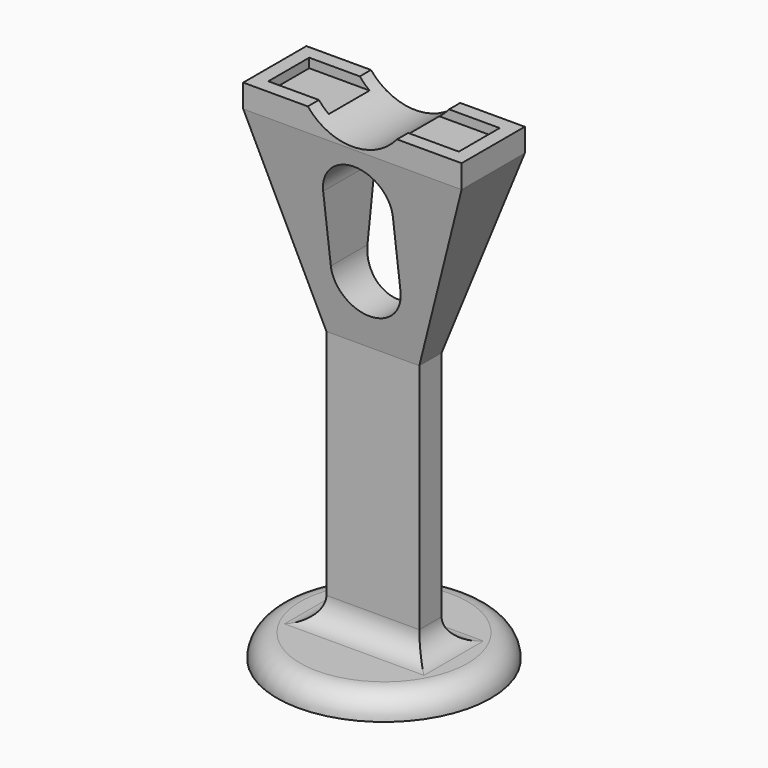
from build123d import *

# Parameters (mm, degrees)
F1_W       = 41
F1_H       = 11
F2_DEPTH   = 3
F1_W_2     = 47
F1_H_2     = 17
F3_DEPTH   = 5
F5_DEPTH   = 17.001
F6_R       = 23
F7_DEPTH   = 5
F8_W       = 20
F8_H       = 6
F9_DEPTH   = 55
F9_FACE_W  = 20
F9_FACE_H  = 6
F3_FACE1_W = 47
F3_FACE1_H = 17
F12_DEPTH  = 25
F13_R      = 4.99999


# Not quite as in the source:
# - a fillet or chamfer is up to 0.001 mm smaller than in the source, because OpenCascade refuses the exact size


with BuildPart() as f2:
    # F1 (on offset) → F2 (new body)
    with BuildSketch(Plane.XY.offset(100)):
        Rectangle(F1_W, F1_H)
    extrude(amount=F2_DEPTH)

    # F1 (on offset) → F3 (join)
    with BuildSketch(Plane.XY.offset(100)):
        Rectangle(F1_W_2, F1_H_2)
        Rectangle(F1_W, F1_H, mode=Mode.SUBTRACT)
    extrude(amount=F3_DEPTH)

    # F4 (on face) → F5 (cut, through all)
    with BuildSketch(Plane.XZ.offset(8.5)):
        with BuildLine():
            Line((9.6046863561, 105), (-9.6046863561, 105))
            ThreePointArc((-9.6046863561, 105), (0, 100.5), (9.6046863561, 105))
        make_face()
    extrude(amount=-F5_DEPTH, mode=Mode.SUBTRACT)



with BuildPart() as f7:
    # F6 (on Top) → F7 (new body)
    with BuildSketch(Plane.XY):
        Circle(F6_R)
    extrude(amount=F7_DEPTH)

    # F8 (on face) → F9 (join)
    with BuildSketch(Plane.XY.offset(5)):
        Rectangle(F8_W, F8_H)
    extrude(amount=F9_DEPTH)


with BuildPart() as f2_1:
    add(f2.part)

    add(f7.part)  # F10 merges F7
    # F9_face (on face) → F10 section 0
    with BuildSketch(Plane.XY.offset(60)):
        Rectangle(F9_FACE_W, F9_FACE_H)
    # F3_face1 (on face) → F10 section 1
    with BuildSketch(Plane(origin=(0, 0, 100), x_dir=(1, 0, 0), z_dir=(0, 0, -1))):
        Rectangle(F3_FACE1_W, F3_FACE1_H)
    loft()

    # F11 (on Front) → F12 (cut, symmetric)
    with BuildSketch(Plane.XZ):
        with BuildLine():
            ThreePointArc((7.5, 89), (0, 96.5), (-7.5, 89))
            Line((-7.5, 89), (-7.5, 74))
            ThreePointArc((-7.5, 74), (0, 66.5), (7.5, 74))
            Line((7.5, 74), (7.5, 89))
        make_face()
    extrude(amount=F12_DEPTH, both=True, mode=Mode.SUBTRACT)

    # F13 (radius 5 in the source; OpenCascade refuses exactly that, so slightly less here)
    f13_edges = [f2_1.edges().sort_by_distance(p)[0] for p in [
        (0, -3, 5),
        (-10, 0, 5),
        (0, 3, 5),
        (10, 0, 5),
        (-23, 0, 5),
    ]]
    fillet(f13_edges, radius=F13_R)


solid = f2_1.part
